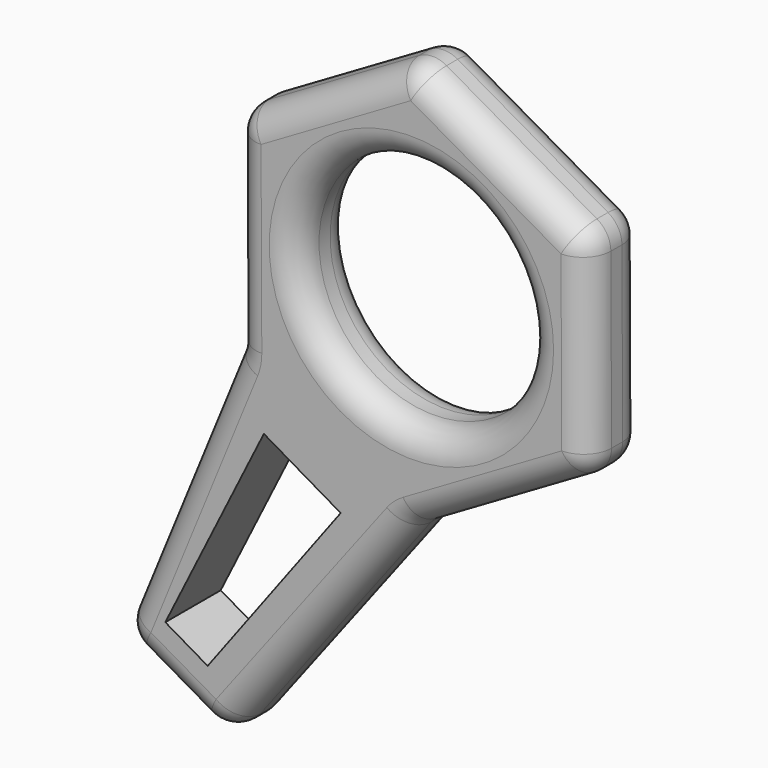
from build123d import *

# Parameters (mm, degrees)
F0_R     = 21.014231477
F1_DEPTH = 12.7
F2_F1_R  = 5.08
F2_F2_R  = 5.08


with BuildPart() as f1:
    # F0 (on Front) → F1 (new body)
    with BuildSketch(Plane.XZ):
        Polygon((0.2339753428, 64.0570990396), (-32.2872099683, 45.1028561744), (-32.132946793, 7.4615621011), (0.5425016933, -11.2254891068), (33.0636870044, 7.7287537585), (32.9094238292, 45.3700478317), align=None)
        with Locations((0.3882385181, 26.4158049664)):
            Circle(F0_R, mode=Mode.SUBTRACT)
        Polygon((0.5425016933, -11.2254891068), (-32.132946793, 7.4615621011), (-53.7858009338, -45.4080328345), (-34.1030090389, -56.7405054673), align=None)
        Polygon((-44.7620823979, -40.694963187), (-26.6759676173, -4.3760748485), (-12.5815442095, -12.5906931584), (-36.9893716799, -45.2251131573), align=None, mode=Mode.SUBTRACT)
    extrude(amount=F1_DEPTH)

    # F2: fillet of radius 5.08 on 22 edges, made by hand

    # F2_f1
    f2_f1_edges = [f1.edges().sort_by_distance(p)[0] for p in [
        (0.5425016933, -6.35, -11.2254891068),
        (-32.132946793, -6.35, 7.4615621011),
    ]]
    fillet(f2_f1_edges, radius=F2_F1_R)

    # F2_f2
    f2_f2_edges = [f1.edges().sort_by_distance(p)[0] for p in [
        (-20.6259929589, -12.7, 26.4158049664),
        (33.0636870044, -6.35, 7.7287537585),
        (17.2393492596, 0, -1.494106292),
        (17.2393492596, -12.7, -1.494106292),
        (32.9094238292, -6.35, 45.3700478317),
        (32.9865554168, 0, 26.5494007951),
        (32.9865554168, -12.7, 26.5494007951),
        (0.2339753428, -6.35, 64.0570990396),
        (16.571699586, 0, 54.7135734357),
        (16.571699586, -12.7, 54.7135734357),
        (-32.2872099683, -6.35, 45.1028561744),
        (-16.0266173128, 0, 54.579977607),
        (-16.0266173128, -12.7, 54.579977607),
        (-53.7858009338, -6.35, -45.4080328345),
        (-43.1509145264, 0, -19.4409186197),
        (-43.1509145264, -12.7, -19.4409186197),
        (-34.1030090389, -6.35, -56.7405054673),
        (-43.9444049864, 0, -51.0742691509),
        (-43.9444049864, -12.7, -51.0742691509),
        (-20.6259929589, 0, 26.4158049664),
        (-32.2306923288, -12.7, 7.4805945272),
        (-32.2306923288, 0, 7.4805945272),
        (0.6083434765, -12.7, -11.2999662173),
        (0.6083434765, 0, -11.2999662173),
    ]]
    fillet(f2_f2_edges, radius=F2_F2_R)


solid = f1.part
